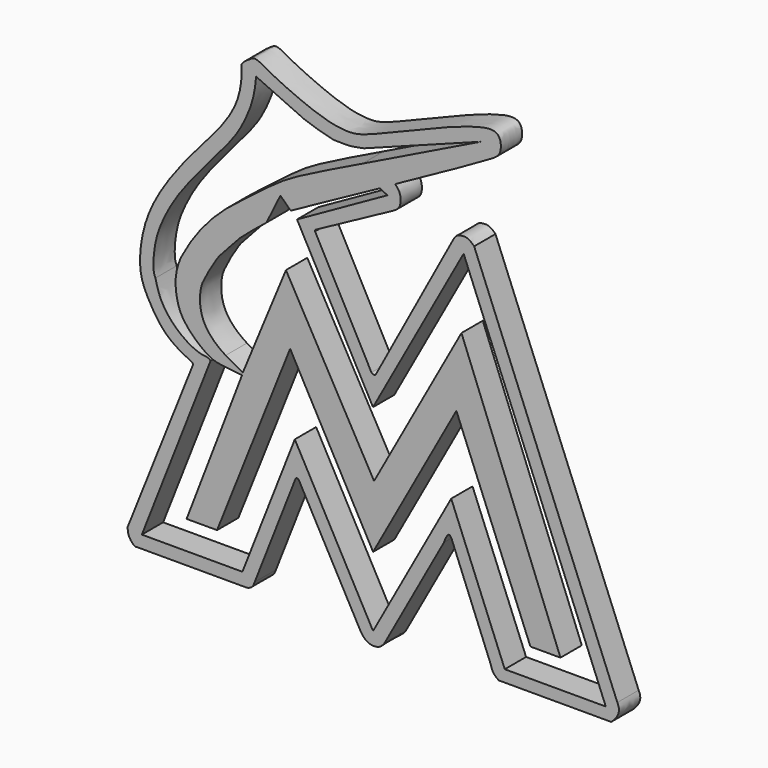
from build123d import *

# Parameters (mm, degrees)
F1_DEPTH = 4
F3_DEPTH = 4


# Not quite as in the source:
# - the program builds the solid bodies; features that only make, move or delete a surface that nothing else refers to are left out


with BuildPart() as f1:
    # F0 (on Front) → F1 (new body)
    with BuildSketch(Plane.XZ):
        Polygon((-19.4217161833, -6.6394530033), (-27.7575291693, -28.3715538681), (-23.1834277511, -28.3715538681), (-12.2142331675, -0.81999955), (0.2424462854, -23.6251421751), (12.7486815966, -0.9048308448), (23.8632653011, -28.4597538413), (28.3766854557, -28.4597538413), (13.5119855407, 9.6240406854), (0.3901409885, -14.2146594537), (-12.8388348967, 9.3706743792), (-19.2233994603, -6.0667619109), (-19.315803546, -6.2901886101), (-19.0307870507, -6.5492987633), align=None)
    extrude(amount=F1_DEPTH)

    # F0 (on Front) → F3 (join)
    with BuildSketch(Plane.XZ):
        with BuildLine():
            add(Edge.make_bspline(
                [(-35.1637251496, -34.5231422063), (-35.2745312626, -34.5561823678), (-35.6035289606, -34.654304467), (-36.6117457532, -33.4166323146), (-36.6023133695, -32.6509350181), (-36.5978814662, -32.2887599468)],
                knots=[0, 0, 0, 0, 0.2111198615, 0.6268416674, 1, 1, 1, 1], degree=3))
            Line((-35.1637251496, -34.5231422063), (-18.7250807702, -34.5231422063))
            add(Edge.make_bspline(
                [(-17.538975038, -33.402744049), (-17.611132101, -33.5982034924), (-17.7255501876, -33.9379030837), (-18.1198933231, -34.3655062286), (-18.5178964655, -34.4823988841), (-18.7250807702, -34.5231422063)],
                knots=[0, 0, 0, 0, 0.3313469636, 0.6551303283, 1, 1, 1, 1], degree=3))
            Line((-17.538975038, -33.402744049), (-11.4031481076, -17.7456413598))
            add(Edge.make_bspline(
                [(-10.749549605, -18.0306378752), (-10.8298087166, -17.9267145736), (-10.9355150168, -17.6876046133), (-11.1533348511, -17.5614089352), (-11.3649684936, -17.6323335618), (-11.4031481076, -17.7456413598)],
                knots=[0, 0, 0, 0, 0.3827269779, 0.6748101929, 1, 1, 1, 1], degree=3))
            Line((-10.749549605, -18.0306378752), (-1.789764151, -34.4338202755))
            add(Edge.make_bspline(
                [(1.9849899689, -35.0782312452), (1.7096466368, -35.4211391418), (1.3050154791, -36.05677829), (-0.6620473159, -36.123537512), (-1.4189460368, -35.0981913004), (-1.789764151, -34.4338202755)],
                knots=[0, 0, 0, 0, 0.2856387916, 0.6247331157, 1, 1, 1, 1], degree=3))
            Line((1.9849899689, -35.0782312452), (10.8746383339, -18.9282409847))
            add(Edge.make_bspline(
                [(12.0244985446, -18.0388428271), (11.9725750544, -17.9490208887), (11.8797340892, -17.78841621), (11.744725143, -17.6291823261), (11.3691565314, -17.67640337), (11.0777840099, -18.4139921669), (10.8746383339, -18.9282409847)],
                knots=[0, 0, 0, 0, 0.2060682504, 0.3684570355, 0.559686611, 1, 1, 1, 1], degree=3))
            Line((12.0244985446, -18.0388428271), (17.9444543715, -32.8427049722))
            add(Edge.make_bspline(
                [(19.1195974171, -34.4750714604), (19.0590878531, -34.4462685115), (18.9069963789, -34.3306804628), (18.1880916185, -33.7704461278), (18.0246763229, -33.1607819226), (17.9444543715, -32.8427049722)],
                knots=[0, 0, 0, 0, 0.2036652656, 0.5896746092, 1, 1, 1, 1], degree=3))
            Line((19.1195974171, -34.4750714604), (35.9913371503, -34.4750714604))
            add(Edge.make_bspline(
                [(36.917551974, -31.6054179477), (37.096636226, -31.9865397753), (37.358811422, -32.7884619292), (36.6453477203, -33.9356747232), (35.9913371503, -34.4750714604)],
                knots=[0, 0, 0, 0, 0.4258250202, 1, 1, 1, 1], degree=3))
            Line((36.917551974, -31.6054179477), (15.4165393649, 21.6992097865))
            add(Edge.make_bspline(
                [(12.2546441238, 21.5262000154), (12.5737046322, 22.0672148588), (12.886276927, 22.4090391583), (13.8326309549, 22.5382735172), (14.5347285525, 22.471159047), (15.1069781666, 22.0141567545), (15.4165393649, 21.6992097865)],
                knots=[0, 0, 0, 0, 0.2748904441, 0.5080982642, 0.721442809, 1, 1, 1, 1], degree=3))
            Line((12.2546441238, 21.5262000154), (0.6201447686, -0.1007694518))
            add(Edge.make_bspline(
                [(0, 0), (0.0863636294, -0.0759495763), (0.2632816512, -0.2315341538), (0.4993266168, -0.1450406271), (0.6201447686, -0.1007694518)],
                knots=[0, 0, 0, 0, 0.4881562014, 1, 1, 1, 1], degree=3))
            Line((0, 0), (-8.4702158347, 15.9015208483))
            add(Edge.make_bspline(
                [(-8.1622106954, 16.276223585), (-8.3447881043, 16.2160024047), (-8.4849828854, 16.110856086), (-8.4702158347, 15.9015208483)],
                knots=[0, 0, 0, 0, 0.4850456749, 0.4850456749, 0.4850456749, 0.4850456749], degree=3))
            Line((-8.1622106954, 16.276223585), (3.1315775122, 22.3828852177))
            add(Edge.make_bspline(
                [(3.5565522512, 26.0707366595), (3.7250692348, 25.8944983199), (4.0768574738, 25.526591336), (4.4162895921, 24.7345286511), (4.3867106206, 23.0702393334), (3.542298202, 22.6078100122), (3.1315775122, 22.3828852177)],
                knots=[0, 0, 0, 0, 0.2048403686, 0.4276152529, 0.721593083, 1, 1, 1, 1], degree=3))
            add(Edge.make_bspline(
                [(-19.4905090892, 34.4106449307), (-19.3913416638, 34.5768098105), (-19.1771283464, 34.8821357986), (-18.2909772268, 35.4649028918), (-17.4167100076, 36.0581049326), (-15.046233937, 34.4869007756), (-8.8847282905, 31.765149045), (-5.5806993412, 30.8516497616), (-2.9868246918, 30.6200128066), (-0.0073204146, 31.2052668466), (16.3641647116, 38.670642674), (19.4600039149, 37.7428738516), (19.5129350415, 35.0531160006), (17.3283449079, 33.686036308), (9.4521634968, 29.2572953328), (3.5565522512, 26.0707366595)],
                knots=[0, 0, 0, 0, 0.0301352733, 0.0712071496, 0.1085985734, 0.1729295184, 0.2794198429, 0.3554207551, 0.415110422, 0.4886293008, 0.6594178969, 0.7227096196, 0.779157198, 0.837654272, 1, 1, 1, 1], degree=3))
            add(Edge.make_bspline(
                [(-26.7625730485, -7.5921593234), (-26.8802814515, -7.4736795432), (-27.1267818843, -7.2257565373), (-27.7274393295, -7.041955029), (-31.0607833825, -5.2827244881), (-33.4673183648, -1.3686976246), (-35.0771704906, 2.0316336914), (-34.4110317157, 8.5701153917), (-31.4521100473, 14.4494388606), (-26.8532177553, 20.3844347406), (-23.0913588106, 24.3697313497), (-19.9077267416, 28.9225104401), (-19.4180184747, 32.4295257558), (-19.4905090892, 34.4106449307)],
                knots=[0, 0, 0, 0, 0.0311082407, 0.0650295367, 0.1496232536, 0.247006076, 0.3333177984, 0.4452947178, 0.5624364483, 0.6851720255, 0.7913099611, 0.8948572122, 1, 1, 1, 1], degree=3))
            Line((-26.7625730485, -7.5921593234), (-36.5978814662, -32.2887599468))
        make_face()
        with BuildLine():
            add(Edge.make_bspline(
                [(-19.4217161833, -6.6394530033), (-19.508625316, -6.6432673623), (-19.8019127291, -6.6566294917), (-20.8924289573, -6.5055145737), (-21.7664551749, -6.406246823), (-22.3774145873, -6.3461085054), (-22.540475484, -6.3254620685)],
                knots=[0, 0, 0, 0, 0.0464939501, 0.1284775828, 0.2166556913, 0.2472364924, 0.2472364924, 0.2472364924, 0.2472364924], degree=3))
            Line((-19.4217161833, -6.6394530033), (-19.0307870507, -6.5492987633))
            Line((-19.0307870507, -6.5492987633), (-19.315803546, -6.2901886101))
            add(Edge.make_bspline(
                [(-21.8946174861, -4.8524995225), (-21.0782101636, -5.3728390923), (-20.1991422317, -5.830401643), (-19.315803546, -6.2901886101)],
                knots=[0.9099002869, 0.9099002869, 0.9099002869, 0.9099002869, 1, 1, 1, 1], degree=3))
            add(Edge.make_bspline(
                [(-15.7669110892, 14.6913326426), (-16.1575708431, 14.3951216587), (-16.9801594317, 13.6529080865), (-19.8434335071, 11.5099121964), (-21.9911810035, 8.7813091437), (-22.9487788, 8.0396329391), (-24.9391358437, 4.6444296479), (-25.8410141184, 2.6584830617), (-25.7767362061, -1.1661814313), (-23.7980017987, -3.5419920665), (-22.300488065, -4.5938167343), (-21.8946174861, -4.8524995225)],
                knots=[0, 0, 0, 0, 0.0799570707, 0.2034389483, 0.3219077837, 0.3946894666, 0.5189098359, 0.61782501, 0.7380766484, 0.8651079121, 0.9099002869, 0.9099002869, 0.9099002869, 0.9099002869], degree=3))
            Line((-15.7669110892, 14.6913326426), (-13.6710712686, 18.9505778253))
            Line((-13.6710712686, 18.9505778253), (-12.1372425929, 17.450094223))
            Line((-12.1372425929, 17.450094223), (1.2483881547, 24.7616254087))
            Line((1.2483881547, 24.7616254087), (2.3965802164, 24.2106570771))
            Line((2.3965802164, 24.2106570771), (-11.1804655804, 16.6029661013))
            Line((-11.1804655804, 16.6029661013), (0.2299634238, -4.4997208142))
            Line((0.2299634238, -4.4997208142), (13.8358174466, 20.2182883726))
            Line((13.8358174466, 20.2182883726), (35.183429718, -32.7060341154))
            Line((35.183429718, -32.7060341154), (20.0139036961, -32.7060341154))
            Line((20.0139036961, -32.7060341154), (11.9725750544, -12.7702274851))
            Line((11.9725750544, -12.7702274851), (0.241156673, -34.082914424))
            Line((0.241156673, -34.082914424), (-11.5100983533, -12.5692319123))
            Line((-11.5100983533, -12.5692319123), (-19.3732271326, -32.6339788733))
            Line((-19.3732271326, -32.6339788733), (-34.4776880647, -32.6339788733))
            Line((-34.4776880647, -32.6339788733), (-24.161764784, -6.3103110171))
            add(Edge.make_bspline(
                [(-24.161764784, -6.3103110171), (-24.2526459585, -6.2458945342), (-24.4218489545, -6.005026647), (-24.7879581492, -6.0032503335), (-26.4467627622, -5.7694302637), (-29.2093356612, -3.9842936163), (-31.0234143453, -1.8115853262), (-31.9290028762, -0.041007341), (-32.2719053848, 1.2774798683), (-32.443283113, 1.9378054652)],
                knots=[0, 0, 0, 0, 0.0692678788, 0.1333973947, 0.2751544883, 0.4850400346, 0.6780474592, 0.8374469779, 1, 1, 1, 1], degree=3))
            add(Edge.make_bspline(
                [(-32.443283113, 1.9378054652), (-32.5460937273, 2.1811675539), (-32.8532037362, 2.9081303087), (-32.6054490494, 6.8315619317), (-31.2056244589, 10.456396718), (-28.545190558, 15.1518389989), (-22.618683209, 21.884807743), (-20.1458962988, 24.9403144345), (-18.6281517866, 27.908594809), (-17.7170611806, 30.3351509939), (-17.4082297731, 32.3915139026), (-17.3176672584, 33.4910062724)],
                knots=[0, 0, 0, 0, 0.0558619343, 0.1669597916, 0.2810807549, 0.415796098, 0.588063338, 0.7035847677, 0.8052847768, 0.8976525607, 1, 1, 1, 1], degree=3))
            add(Edge.make_bspline(
                [(-17.3176672584, 33.4910062724), (-17.221630037, 33.4597220725), (-16.9720207923, 33.3469005033), (-13.5430734754, 31.8596596856), (-10.0203260912, 29.9973066976), (-7.1406603696, 29.2607063143), (-5.6896028796, 28.9016544729)],
                knots=[0, 0, 0, 0, 0.0862425306, 0.3671206301, 0.682503877, 1, 1, 1, 1], degree=3))
            add(Edge.make_bspline(
                [(-5.6896028796, 28.9016544729), (-4.9036243336, 28.8691385408), (-3.3396702778, 28.8042656638), (-1.8322599185, 29.1262884352), (-1.0824227938, 29.2862113565)],
                knots=[0, 0, 0, 0, 0.5025756584, 1, 1, 1, 1], degree=3))
            Line((-1.0824227938, 29.2862113565), (16.3887608796, 35.8408540487))
            Line((16.3887608796, 35.8408540487), (-1.3610265687, 27.1718096203))
            add(Edge.make_bspline(
                [(-28.3569605203, 6.3584583539), (-28.2130936728, 6.6411128815), (-27.8271836576, 7.4023465501), (-25.7733867324, 10.6560215753), (-22.0445767964, 14.6239494535), (-17.4960241663, 17.781024568), (-12.7864597899, 21.8271717018), (-5.5598486203, 25.0804798141), (-1.3610265687, 27.1718096203)],
                knots=[0, 0, 0, 0, 0.0755576656, 0.2159621836, 0.3892077102, 0.5588631934, 0.7384412181, 1, 1, 1, 1], degree=3))
            add(Edge.make_bspline(
                [(-22.540475484, -6.3254620685), (-22.9495394006, -6.2736672328), (-24.22734435, -6.0317724791), (-26.6434003655, -4.1641087229), (-28.453733366, -2.0639095463), (-29.2248130286, 0.0009913676), (-29.6205864439, 3.0557923807), (-28.9095027831, 5.3913160175), (-28.3569605203, 6.3584583539)],
                knots=[0.2472364924, 0.2472364924, 0.2472364924, 0.2472364924, 0.3239532439, 0.4674432485, 0.5991747745, 0.7144941387, 0.852062496, 1, 1, 1, 1], degree=3))
        make_face(mode=Mode.SUBTRACT)
    extrude(amount=F3_DEPTH)


solid = f1.part
